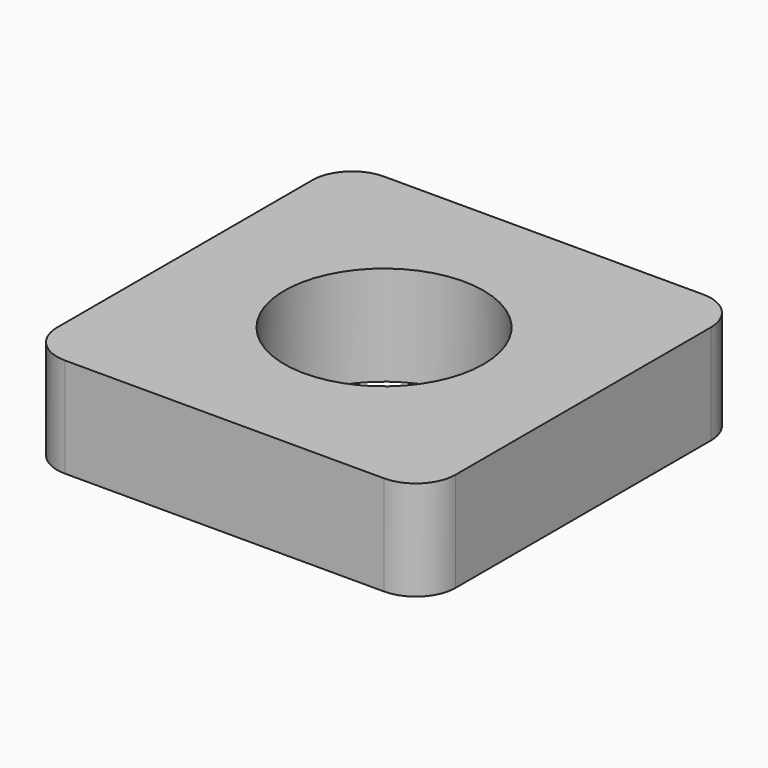
from build123d import *

# Parameters (mm, degrees)
F0_W     = 20
F0_H     = 20
F0_R     = 5
F1_DEPTH = 5
F2_R     = 2


# Not quite as in the source:
# - a feature of the source that left no trace in its solid (it failed there, or was rolled back) is left out


with BuildPart() as f1:
    # F0 (on Top) → F1 (new body)
    with BuildSketch(Plane.XY):
        Rectangle(F0_W, F0_H)
        Circle(F0_R, mode=Mode.SUBTRACT)
    extrude(amount=F1_DEPTH)

    # F2
    f2_edges = [f1.edges().sort_by_distance(p)[0] for p in [
        (-10, -10, 2.5),
        (10, -10, 2.5),
        (10, 10, 2.5),
        (-10, 10, 2.5),
    ]]
    fillet(f2_edges, radius=F2_R)


solid = f1.part
